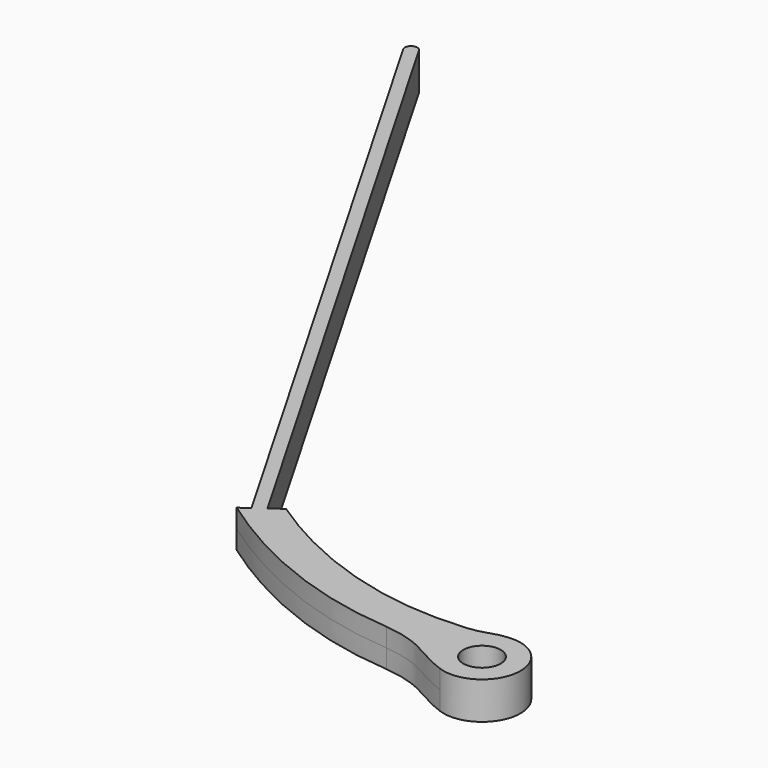
from build123d import *

# Parameters (mm, degrees)
F1_DEPTH = 1.5
F2_R     = 1.5
F3_DEPTH = 25


# Not quite as in the source:
# - the dataset's text gives a spline's control points without its knots; the knots are read off the source's solid


with BuildPart() as f1:
    # F0 (on Top) → F1 (new body, symmetric)
    with BuildSketch(Plane.XY):
        with BuildLine():
            add(Edge.make_bspline(
                [(-7.2290541015, -0.5527675977), (-3.9967772573, -0.8917449116), (-3.2988634653, -2.0894490401), (-1.0464995032, -2.9017509308)],
                knots=[0, 0, 0, 0, 6.6137511338, 6.6137511338, 6.6137511338, 6.6137511338], degree=3))
            ThreePointArc((-1.0464995032, -2.9017509308), (3.0587935975, -0.3988751709), (-0.2673646533, 3.0730824617))
            add(Edge.make_bspline(
                [(-3.0769753559, 2.4563793473), (-1.7409748989, 2.5984151431), (-1.6058379576, 2.9566324623), (-0.2673646533, 3.0730824617)],
                knots=[0, 0, 0, 0, 2.876497007, 2.876497007, 2.876497007, 2.876497007], degree=3))
            add(Edge.make_bspline(
                [(-3.0769753559, 2.4563793473), (-5.7816746579, 2.1906947352), (-11.4426782467, 2.6135423344), (-17.8801982674, 5.2791288997), (-21.4653904829, 7.5502048837), (-22.1168282691, 7.9895307861)],
                knots=[0.005973262, 0.005973262, 0.005973262, 0.005973262, 0.125, 0.25, 0.277850749, 0.277850749, 0.277850749, 0.277850749], degree=3))
            Line((-22.1168282691, 7.9895307861), (-23.0633222923, 7.3125738031))
            Line((-23.0633222923, 7.3125738031), (-54.4799332581, 61.7749325905))
            ThreePointArc((-54.4799332581, 61.7749325905), (-55.1628772285, 61.9582016093), (-55.3461462473, 61.2752576388))
            Line((-55.3461462473, 61.2752576388), (-23.8805872256, 6.7280448046))
            Line((-23.8805872256, 6.7280448046), (-24.6317860127, 6.1907680209))
            add(Edge.make_bspline(
                [(-7.2290541015, -0.5527675977), (-8.7909293011, -0.4393198693), (-13.6136774425, 0.3217510425), (-19.4562298082, 2.7561257866), (-23.6206363974, 5.4709704249), (-24.6317860127, 6.1907680209)],
                knots=[0.064829406, 0.064829406, 0.064829406, 0.064829406, 0.125, 0.25, 0.290542228, 0.290542228, 0.290542228, 0.290542228], degree=3))
        make_face()
    extrude(amount=F1_DEPTH, both=True)

    # F2 (on face) → F3 (cut)
    with BuildSketch(Plane(origin=(0, 0, -1.5), x_dir=(1, 0, 0), z_dir=(0, 0, -1))):
        Circle(F2_R)
    extrude(amount=-F3_DEPTH, mode=Mode.SUBTRACT)


solid = f1.part
